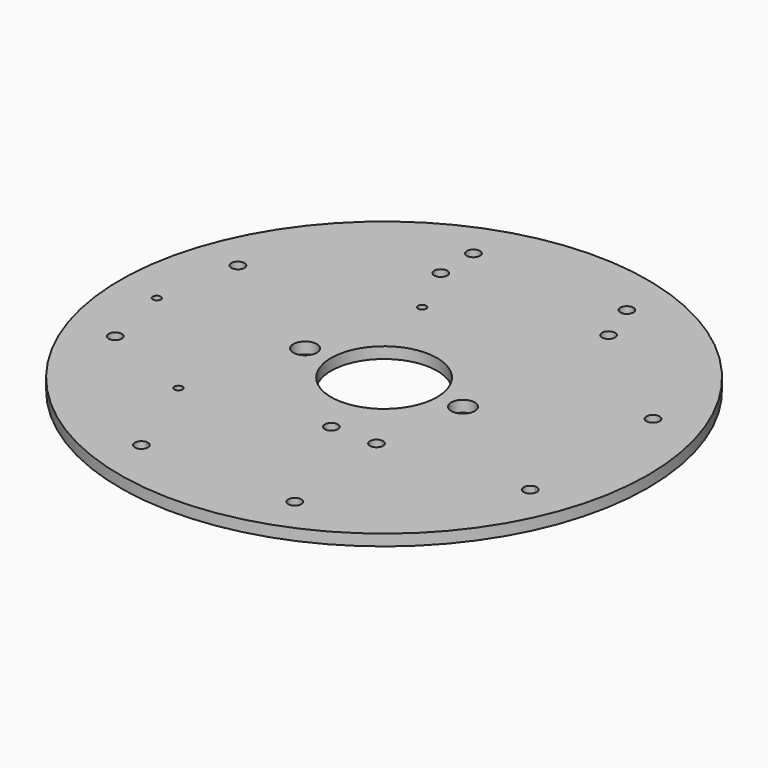
from build123d import *

# Parameters (mm, degrees)
F0_R            = 74.295
F1_DEPTH        = 3.175
F2_R            = 1.8542
F3_DEPTH        = 3.176
F3_COPIES_COUNT = 4
F4_R            = 14.9225
F4_R_2          = 3.302
F5_DEPTH        = 3.176
F6_R            = 1.8415
F7_DEPTH        = 3.176
F8_R            = 1.1303
F9_DEPTH        = 3.176


# Not quite as in the source:
# - a pattern or mirror of a feature is missing from the dataset's text; its kind, count and spacing are read off the source's solid


with BuildPart() as f1:
    # F0 (on Top) → F1 (new body)
    with BuildSketch(Plane.XY):
        Circle(F0_R)
    extrude(amount=F1_DEPTH)

    # F2 (on face) → F3 (cut, through all)
    with BuildSketch(Plane.XY.offset(3.175)):
        with BuildLine():
            ThreePointArc((-58.42, 19.7358), (-57.1088826063, 20.2788826063), (-56.5658, 21.59))
            ThreePointArc((-56.5658, 21.59), (-59.7311173937, 22.9011173937), (-58.42, 19.7358))
        make_face()
        with Locations((-58.42, -21.59)):
            Circle(F2_R)
    f3 = extrude(amount=-F3_DEPTH, mode=Mode.SUBTRACT)

    # F3_copies: F3 ×4 about axis
    f3_copies_axis = Axis((0, 0, 0), (0, 0, 1))
    for i in range(1, F3_COPIES_COUNT):
        add(f3.rotate(f3_copies_axis, i * 360 / F3_COPIES_COUNT), mode=Mode.SUBTRACT)

    # F4 (on face) → F5 (cut, through all)
    with BuildSketch(Plane.XY.offset(3.175)):
        Circle(F4_R)
        with Locations((-22.225, 0)):
            Circle(F4_R_2)
        with Locations((22.225, 0)):
            Circle(F4_R_2)
    extrude(amount=-F5_DEPTH, mode=Mode.SUBTRACT)

    # F6 (on face) → F7 (cut, through all)
    with BuildSketch(Plane.XY.offset(3.175)):
        with Locations((-21.330000012, 46.603412)):
            Circle(F6_R)
        with Locations((25.913999988, 46.603412)):
            Circle(F6_R)
        with Locations((5.593999988, -25.532588)):
            Circle(F6_R)
        with Locations((18.293999988, -25.532588)):
            Circle(F6_R)
    extrude(amount=-F7_DEPTH, mode=Mode.SUBTRACT)

    # F8 (on face) → F9 (cut, through all)
    with BuildSketch(Plane.XY.offset(3.175)):
        with Locations((-14.3844060319, 31.369)):
            Circle(F8_R)
        with Locations((-62.6444060319, -1.651)):
            Circle(F8_R)
        with Locations((-32.1644060319, -32.131)):
            Circle(F8_R)
    extrude(amount=-F9_DEPTH, mode=Mode.SUBTRACT)


solid = f1.part
